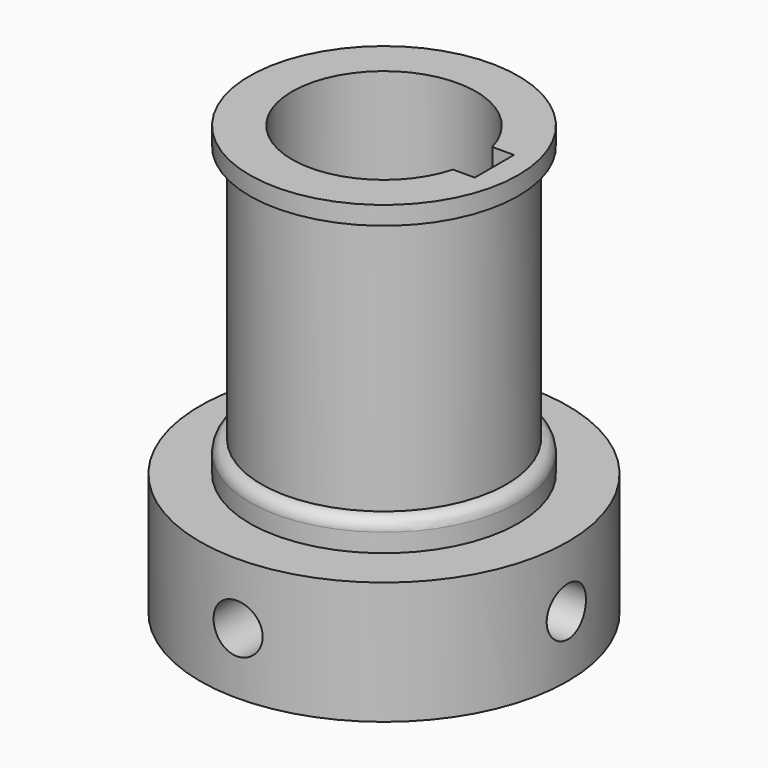
from build123d import *

# Parameters (mm, degrees)
F0_R           = 30
F1_DEPTH       = 20
F2_R           = 21.9
F3_DEPTH       = 5
F4_R           = 20
F5_DEPTH       = 42
F6_R           = 21.9
F7_DEPTH       = 3
F10_DEPTH      = 75
F11_R          = 4
F12_DEPTH      = 100
F12_DEPTH_BACK = 100
F13_R          = 4
F14_DEPTH      = 100
F14_DEPTH_BACK = 100


# Not quite as in the source:
# - a fillet or chamfer that OpenCascade refuses, or shapes differently, is made with other operations: its cross-section is extruded or revolved along the edge and cut away or added


with BuildPart() as f1:
    # F0 (on Top) → F1 (new body)
    with BuildSketch(Plane.XY):
        Circle(F0_R)
    extrude(amount=F1_DEPTH)

    # F2 (on face) → F3 (join)
    with BuildSketch(Plane.XY.offset(20)):
        Circle(F2_R)
    extrude(amount=F3_DEPTH)

    # F4 (on face) → F5 (join)
    with BuildSketch(Plane.XY.offset(25)):
        Circle(F4_R)
    extrude(amount=F5_DEPTH)

    # F6 (on face) → F7 (join)
    with BuildSketch(Plane.XY.offset(67)):
        Circle(F6_R)
    extrude(amount=F7_DEPTH)

    # F8: fillet of radius 2 on 1 edges, made by hand

    # F8_s1 → F8_t2 (revolve, cut)
    with BuildSketch(Plane.XZ):
        with BuildLine():
            ThreePointArc((20, 25), (21.3491376746, 24.3809064397), (21.9, 23.0025015645))
            Line((21.9, 23.0025015645), (21.9, 25))
            Line((21.9, 25), (20, 25))
        make_face()
    revolve(axis=Axis((0, 0, 25), (0, 0, 1)), mode=Mode.SUBTRACT)

    # F9 (on face) → F10 (cut)
    with BuildSketch(Plane.XY.offset(70)):
        with BuildLine():
            Line((18, 4), (14.4568322948, 4))
            ThreePointArc((14.4568322948, 4), (-2.0183552187, 14.8635877974), (-15, 0))
            Line((-15, 0), (0, 0))
            Line((0, 0), (15, 0))
            Line((15, 0), (18, 0))
            Line((18, 0), (18, 4))
        make_face()
        with BuildLine():
            Line((0, 0), (-15, 0))
            ThreePointArc((-15, 0), (-2.0183552187, -14.8635877974), (14.4568322948, -4))
            Line((14.4568322948, -4), (18, -4))
            Line((18, -4), (18, 0))
            Line((18, 0), (15, 0))
            Line((15, 0), (0, 0))
        make_face()
    extrude(amount=-F10_DEPTH, mode=Mode.SUBTRACT)

    # F11 (on Right) → F12 (cut, two sides)
    with BuildSketch(Plane.YZ) as f12_sk:
        with Locations((0, 10)):
            Circle(F11_R)
    extrude(amount=F12_DEPTH, mode=Mode.SUBTRACT)
    extrude(f12_sk.sketch, amount=-F12_DEPTH_BACK, mode=Mode.SUBTRACT)

    # F13 (on Front) → F14 (cut, two sides)
    with BuildSketch(Plane.XZ) as f14_sk:
        with Locations((0, 10)):
            Circle(F13_R)
    extrude(amount=-F14_DEPTH, mode=Mode.SUBTRACT)
    extrude(f14_sk.sketch, amount=F14_DEPTH_BACK, mode=Mode.SUBTRACT)


solid = f1.part
